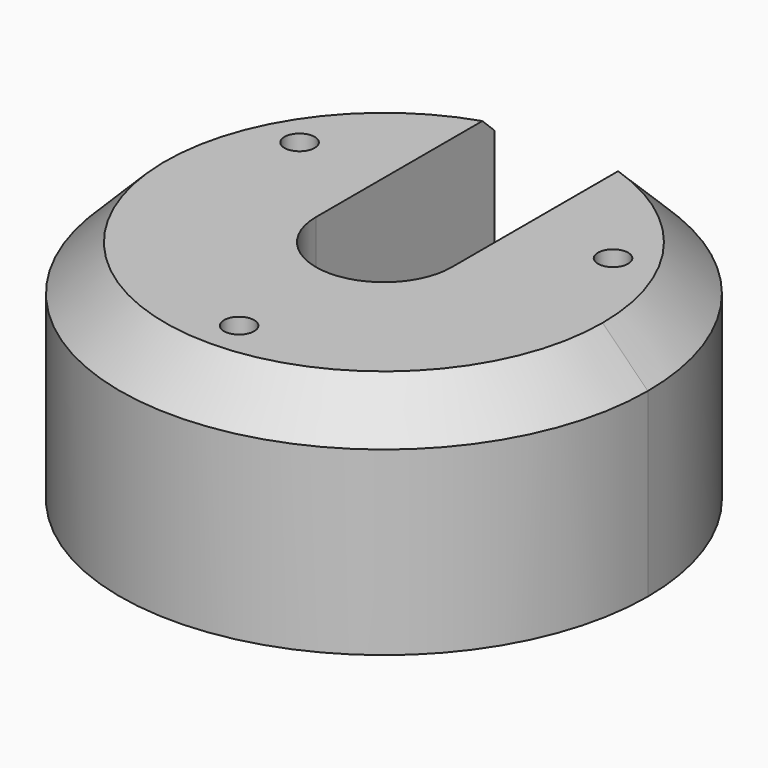
from build123d import *

# Parameters (mm, degrees)
F0_R        = 1
F1_DEPTH    = 15
F2_SIZE     = 3
F3_T1_DEPTH = 23.4240423609


# Not quite as in the source:
# - a fillet or chamfer that OpenCascade refuses, or shapes differently, is made with other operations: its cross-section is extruded or revolved along the edge and cut away or added


with BuildPart() as f1:
    # F0 (on Top) → F1 (new body)
    with BuildSketch(Plane.XY):
        with BuildLine():
            ThreePointArc((-4.5, 16.9115345253), (-10.6653645039, -13.8744369255), (17.5, 0))
            ThreePointArc((17.5, 0), (13.8744369255, 10.6653645039), (4.5, 16.9115345253))
            Line((4.5, 16.9115345253), (4.5, 0))
            ThreePointArc((4.5, 0), (0, -4.5), (-4.5, 0))
            Line((-4.5, 0), (-4.5, 16.9115345253))
        make_face()
        with Locations((0, -12)):
            Circle(F0_R, mode=Mode.SUBTRACT)
        with Locations((-10.3923048454, 6)):
            Circle(F0_R, mode=Mode.SUBTRACT)
        with Locations((10.3923048454, 6)):
            Circle(F0_R, mode=Mode.SUBTRACT)
    extrude(amount=F1_DEPTH)

    # F2
    f2_edges = [f1.edges().sort_by_distance(p)[0] for p in [
        (-10.665365, -13.874437, 15),
        (13.874437, 10.665365, 15),
    ]]
    chamfer(f2_edges, length=F2_SIZE)

    # F3: chamfer of 2 on 2 edges, made by hand

    # F3_s2 → F3_t1 (cut)
    with BuildSketch(Plane.XY.offset(-5.7120211805)):
        with BuildLine():
            Line((-6.685306539, 16.244612427), (-4.4335898165, 14.7321955637))
            Line((-4.4335898165, 14.7321955637), (-4.3935898165, 14.7321955637))
            ThreePointArc((-4.3935898165, 14.7321955637), (-4.46, 15.8218650445), (-4.46, 16.9115345253))
            Line((-4.46, 16.9115345253), (-4.5102857143, 16.9501894613))
            ThreePointArc((-4.5102857143, 16.9501894613), (-5.6067154961, 16.6197575598), (-6.700435445, 16.2816410133))
            Line((-6.700435445, 16.2816410133), (-6.685306539, 16.244612427))
        make_face()
        with BuildLine():
            Line((4.4335898165, 14.7321955637), (6.685306539, 16.244612427))
            Line((6.685306539, 16.244612427), (6.700435445, 16.2816410133))
            ThreePointArc((6.700435445, 16.2816410133), (5.6067154961, 16.6197575598), (4.5102857143, 16.9501894613))
            Line((4.5102857143, 16.9501894613), (4.46, 16.9115345253))
            ThreePointArc((4.46, 16.9115345253), (4.46, 15.8218650445), (4.3935898165, 14.7321955637))
            Line((4.3935898165, 14.7321955637), (4.4335898165, 14.7321955637))
        make_face()
    extrude(amount=F3_T1_DEPTH, mode=Mode.SUBTRACT)


solid = f1.part
